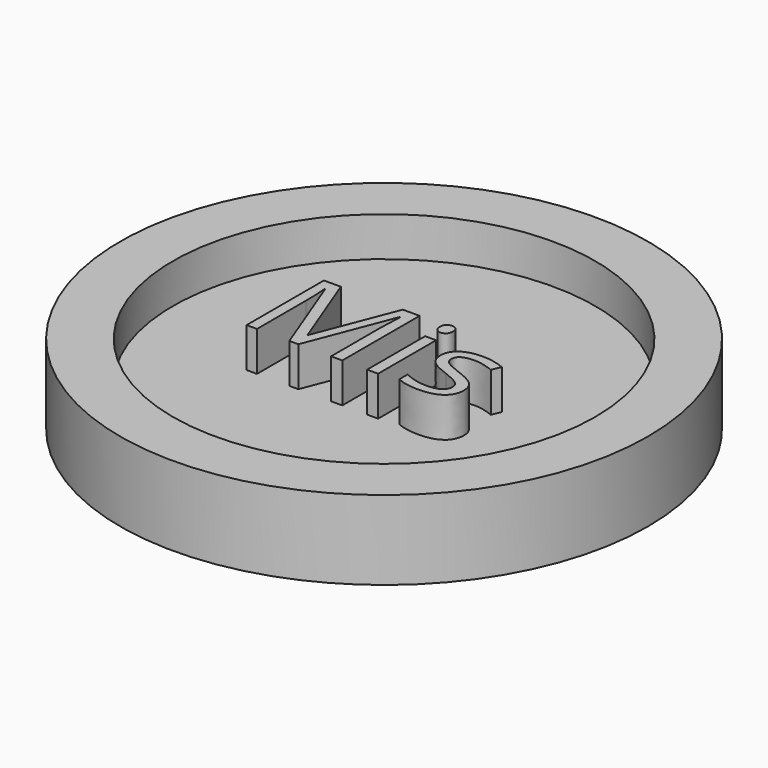
from build123d import *

# Parameters (mm, degrees)
F0_R         = 10
F0_R_2       = 8
F0_TEXT_SIZE = 5.1285398917
F1_DEPTH     = 3
F0_W         = 0.4158925318
F0_H         = 2.7445701764
F2_DEPTH     = 1.5


# Not quite as in the source:
# - Text() gives the source's letters only with a copy of the font that has no kerning and outlines rounded to 1/6400 em; it was checked with that copy


with BuildPart() as f1:
    # F0 (on Top) → F1 (new body)
    with BuildSketch(Plane.XY):
        with Locations((-7.1337355665, 1.846274361)):
            Circle(F0_R)
        with Locations((-7.1337355665, 1.846274361)):
            Circle(F0_R_2, mode=Mode.SUBTRACT)
        with Locations((-11.3691883162, 0)):
            Text('Mis', F0_TEXT_SIZE, font='Open Sans', text_align=(TextAlign.LEFT, TextAlign.BOTTOM))
    extrude(amount=F1_DEPTH)

    # F0 (on Top) → F2 (join)
    with BuildSketch(Plane.XY):
        with Locations((-7.1337355665, 1.846274361)):
            Circle(F0_R_2)
        with BuildLine():
            Line((-8.902681162, 0), (-9.2456522673, 0))
            Line((-9.2456522673, 0), (-10.4877205223, 3.2454041502))
            Line((-10.4877205223, 3.2454041502), (-10.5077538812, 3.2454041502))
            add(Edge.make_bspline(
                [(-10.5077538812, 3.2454041502), (-10.4724951695, 2.859962324), (-10.4724951695, 2.3286776446)],
                knots=[0, 0, 0, 1, 1, 1], degree=2))
            Line((-10.4724951695, 2.3286776446), (-10.4724951695, 0))
            Line((-10.4724951695, 0), (-10.8659503393, 0))
            Line((-10.8659503393, 0), (-10.8659503393, 3.6612966821))
            Line((-10.8659503393, 3.6612966821), (-10.2248828528, 3.6612966821))
            Line((-10.2248828528, 3.6612966821), (-9.0653520367, 0.6410674865))
            Line((-9.0653520367, 0.6410674865), (-9.0453186777, 0.6410674865))
            Line((-9.0453186777, 0.6410674865), (-7.8761718493, 3.6612966821))
            Line((-7.8761718493, 3.6612966821), (-7.239912369, 3.6612966821))
            Line((-7.239912369, 3.6612966821), (-7.239912369, 0))
            Line((-7.239912369, 0), (-7.6654209131, 0))
            Line((-7.6654209131, 0), (-7.6654209131, 2.3591283502))
            add(Edge.make_bspline(
                [(-7.6654209131, 2.3591283502), (-7.6654209131, 2.7646035354), (-7.6301622014, 3.2405961441)],
                knots=[0, 0, 0, 1, 1, 1], degree=2))
            Line((-7.6301622014, 3.2405961441), (-7.6501955603, 3.2405961441))
            Line((-7.6501955603, 3.2405961441), (-8.902681162, 0))
        make_face(mode=Mode.SUBTRACT)
        with Locations((-6.0903982323, 1.3722850882)):
            Rectangle(F0_W, F0_H, mode=Mode.SUBTRACT)
        with BuildLine():
            add(Edge.make_bspline(
                [(-3.4023221281, 1.2020015371), (-3.2308365755, 1.0217013066), (-3.2308365755, 0.7484462904)],
                knots=[0, 0, 0, 1, 1, 1], degree=2))
            add(Edge.make_bspline(
                [(-3.2308365755, 0.7484462904), (-3.2308365755, 0.3654084673), (-3.516111607, 0.1574622014)],
                knots=[0, 0, 0, 1, 1, 1], degree=2))
            add(Edge.make_bspline(
                [(-3.516111607, 0.1574622014), (-3.8013866385, -0.0504840646), (-4.3174459651, -0.0504840646)],
                knots=[0, 0, 0, 1, 1, 1], degree=2))
            add(Edge.make_bspline(
                [(-4.3174459651, -0.0504840646), (-4.8631546629, -0.0504840646), (-5.1684630533, 0.1226041568)],
                knots=[0, 0, 0, 1, 1, 1], degree=2))
            Line((-5.1684630533, 0.1226041568), (-5.1684630533, 0.508045983))
            add(Edge.make_bspline(
                [(-5.1684630533, 0.508045983), (-4.9705334669, 0.4078791883), (-4.7441565107, 0.3505837817)],
                knots=[0, 0, 0, 1, 1, 1], degree=2))
            add(Edge.make_bspline(
                [(-4.7441565107, 0.3505837817), (-4.5177795546, 0.2932883751), (-4.3070286184, 0.2932883751)],
                knots=[0, 0, 0, 1, 1, 1], degree=2))
            add(Edge.make_bspline(
                [(-4.3070286184, 0.2932883751), (-3.981686869, 0.2932883751), (-3.8065953118, 0.3970611744)],
                knots=[0, 0, 0, 1, 1, 1], degree=2))
            add(Edge.make_bspline(
                [(-3.8065953118, 0.3970611744), (-3.6315037546, 0.5008339738), (-3.6315037546, 0.713988913)],
                knots=[0, 0, 0, 1, 1, 1], degree=2))
            add(Edge.make_bspline(
                [(-3.6315037546, 0.713988913), (-3.6315037546, 0.8742557847), (-3.7701345985, 0.9880452635)],
                knots=[0, 0, 0, 1, 1, 1], degree=2))
            add(Edge.make_bspline(
                [(-3.7701345985, 0.9880452635), (-3.9087654424, 1.1018347424), (-4.3126379589, 1.2572936078)],
                knots=[0, 0, 0, 1, 1, 1], degree=2))
            add(Edge.make_bspline(
                [(-4.3126379589, 1.2572936078), (-4.6956757821, 1.3999311236), (-4.8571446552, 1.5065085932)],
                knots=[0, 0, 0, 1, 1, 1], degree=2))
            add(Edge.make_bspline(
                [(-4.8571446552, 1.5065085932), (-5.0186135284, 1.6130860628), (-5.0975449627, 1.7481109021)],
                knots=[0, 0, 0, 1, 1, 1], degree=2))
            add(Edge.make_bspline(
                [(-5.0975449627, 1.7481109021), (-5.1764763969, 1.8831357415), (-5.1764763969, 2.0706479813)],
                knots=[0, 0, 0, 1, 1, 1], degree=2))
            add(Edge.make_bspline(
                [(-5.1764763969, 2.0706479813), (-5.1764763969, 2.4064070773), (-4.9032213808, 2.6007306591)],
                knots=[0, 0, 0, 1, 1, 1], degree=2))
            add(Edge.make_bspline(
                [(-4.9032213808, 2.6007306591), (-4.6299663647, 2.795054241), (-4.1547750904, 2.795054241)],
                knots=[0, 0, 0, 1, 1, 1], degree=2))
            add(Edge.make_bspline(
                [(-4.1547750904, 2.795054241), (-3.7116371904, 2.795054241), (-3.2877313149, 2.6147540104)],
                knots=[0, 0, 0, 1, 1, 1], degree=2))
            Line((-3.2877313149, 2.6147540104), (-3.4359781712, 2.2765909113))
            add(Edge.make_bspline(
                [(-3.4359781712, 2.2765909113), (-3.8486653656, 2.4464737952), (-4.1844244616, 2.4464737952)],
                knots=[0, 0, 0, 1, 1, 1], degree=2))
            add(Edge.make_bspline(
                [(-4.1844244616, 2.4464737952), (-4.4801168398, 2.4464737952), (-4.6303670319, 2.3539196769)],
                knots=[0, 0, 0, 1, 1, 1], degree=2))
            add(Edge.make_bspline(
                [(-4.6303670319, 2.3539196769), (-4.780617224, 2.2613655585), (-4.780617224, 2.0986946838)],
                knots=[0, 0, 0, 1, 1, 1], degree=2))
            add(Edge.make_bspline(
                [(-4.780617224, 2.0986946838), (-4.780617224, 1.9881105424), (-4.7241231518, 1.9107817768)],
                knots=[0, 0, 0, 1, 1, 1], degree=2))
            add(Edge.make_bspline(
                [(-4.7241231518, 1.9107817768), (-4.6676290796, 1.8334530113), (-4.5426209197, 1.763336255)],
                knots=[0, 0, 0, 1, 1, 1], degree=2))
            add(Edge.make_bspline(
                [(-4.5426209197, 1.763336255), (-4.4176127598, 1.6932194986), (-4.0618203048, 1.5601979952)],
                knots=[0, 0, 0, 1, 1, 1], degree=2))
            add(Edge.make_bspline(
                [(-4.0618203048, 1.5601979952), (-3.5738076808, 1.3823017677), (-3.4023221281, 1.2020015371)],
                knots=[0, 0, 0, 1, 1, 1], degree=2))
        make_face(mode=Mode.SUBTRACT)
        with BuildLine():
            add(Edge.make_bspline(
                [(-6.2634864537, 3.2790601933), (-6.33360321, 3.3479749481), (-6.33360321, 3.4882084607)],
                knots=[0, 0, 0, 1, 1, 1], degree=2))
            add(Edge.make_bspline(
                [(-6.33360321, 3.4882084607), (-6.33360321, 3.6308459765), (-6.2634864537, 3.6973567282)],
                knots=[0, 0, 0, 1, 1, 1], degree=2))
            add(Edge.make_bspline(
                [(-6.2634864537, 3.6973567282), (-6.1933696973, 3.7638674799), (-6.0875935621, 3.7638674799)],
                knots=[0, 0, 0, 1, 1, 1], degree=2))
            add(Edge.make_bspline(
                [(-6.0875935621, 3.7638674799), (-5.9874267673, 3.7638674799), (-5.9149060079, 3.6961547266)],
                knots=[0, 0, 0, 1, 1, 1], degree=2))
            add(Edge.make_bspline(
                [(-5.9149060079, 3.6961547266), (-5.8423852485, 3.6284419734), (-5.8423852485, 3.4882084607)],
                knots=[0, 0, 0, 1, 1, 1], degree=2))
            add(Edge.make_bspline(
                [(-5.8423852485, 3.4882084607), (-5.8423852485, 3.3479749481), (-5.9149060079, 3.2790601933)],
                knots=[0, 0, 0, 1, 1, 1], degree=2))
            add(Edge.make_bspline(
                [(-5.9149060079, 3.2790601933), (-5.9874267673, 3.2101454385), (-6.0875935621, 3.2101454385)],
                knots=[0, 0, 0, 1, 1, 1], degree=2))
            add(Edge.make_bspline(
                [(-6.0875935621, 3.2101454385), (-6.1933696973, 3.2101454385), (-6.2634864537, 3.2790601933)],
                knots=[0, 0, 0, 1, 1, 1], degree=2))
        make_face(mode=Mode.SUBTRACT)
    extrude(amount=F2_DEPTH)


solid = f1.part
